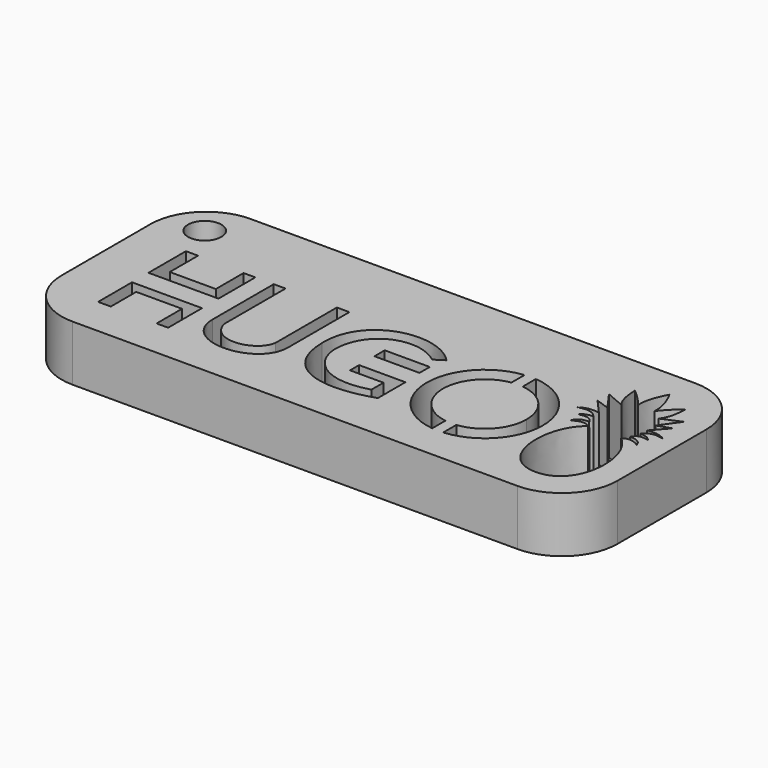
from build123d import *

# Parameters (mm, degrees)
F0_R     = 1.5
F0_W     = 3.6842799746
F0_H     = 1.051153522
F1_DEPTH = 5
F3_DEPTH = 25
F2_W     = 3.6842799746
F2_H     = 1.051153522
F4_SCALE = 1.1
F8_DEPTH = 5


with BuildPart() as f1:
    # F0 (on Top) → F1 (new body)
    with BuildSketch(Plane.XY):
        with BuildLine():
            Line((19.5023587838, 5.8855334138), (-19.8380679384, 5.8855334138))
            ThreePointArc((-19.8380679384, 5.8855334138), (-23.3736018443, 4.4210673197), (-24.8380679384, 0.8855334138))
            Line((-24.8380679384, 0.8855334138), (-24.8380679384, -9.1144665862))
            ThreePointArc((-24.8380679384, -9.1144665862), (-23.3736018443, -12.6500004921), (-19.8380679384, -14.1144665862))
            Line((-19.8380679384, -14.1144665862), (19.8321454227, -14.1144665862))
            Line((19.8321454227, -14.1144665862), (19.8321454227, -11.658272632))
            add(Edge.make_bspline(
                [(18.3578059077, -3.9089675993), (15.9339979291, -5.7451855391), (16.1109714375, -11.6508233578), (19.8321454227, -11.658272632)],
                knots=[0, 0, 0, 0, 7.8883081517, 7.8883081517, 7.8883081517, 7.8883081517], degree=3))
            add(Edge.make_bspline(
                [(18.3578059077, -3.9089675993), (18.0898513645, -3.72885447), (17.704680562, -3.4674885683), (16.8380476534, -4.0177325718)],
                knots=[0, 0, 0, 0, 1.5236452903, 1.5236452903, 1.5236452903, 1.5236452903], degree=3))
            add(Edge.make_bspline(
                [(16.8380476534, -4.0177325718), (16.9854741544, -3.645024728), (17.2194819897, -3.3108589705), (17.980273813, -3.3471628558)],
                knots=[0, 0, 0, 0, 1.3245166453, 1.3245166453, 1.3245166453, 1.3245166453], degree=3))
            add(Edge.make_bspline(
                [(17.980273813, -3.3471628558), (17.7715364844, -2.8870156966), (17.4005404115, -2.7581979521), (16.6894663125, -2.9488482978)],
                knots=[0, 0, 0, 0, 1.3508658299, 1.3508658299, 1.3508658299, 1.3508658299], degree=3))
            add(Edge.make_bspline(
                [(16.6894663125, -2.9488482978), (16.9780198485, -2.5830056984), (17.2820296139, -2.5572420564), (17.709704116, -2.5057150051)],
                knots=[0, 0, 0, 0, 1.1123184305, 1.1123184305, 1.1123184305, 1.1123184305], degree=3))
            add(Edge.make_bspline(
                [(17.709704116, -2.5057150051), (17.3335559666, -2.0625817124), (16.911033541, -1.8873894587), (15.9629341215, -2.1450251807)],
                knots=[0, 0, 0, 0, 1.7836206332, 1.7836206332, 1.7836206332, 1.7836206332], degree=3))
            add(Edge.make_bspline(
                [(15.9629341215, -2.1450251807), (16.4724756032, -1.8160737818), (16.910193488, -1.7090764595), (17.6636241376, -1.833897084)],
                knots=[0, 0, 0, 0, 1.7289150423, 1.7289150423, 1.7289150423, 1.7289150423], degree=3))
            Line((17.6636241376, -1.833897084), (16.4479874074, -0.4642672138))
            Line((16.4479874074, -0.4642672138), (17.6636241376, -0.8728023386))
            Line((17.6636241376, -0.8728023386), (16.4674408734, 0.80024614))
            Line((16.4674408734, 0.80024614), (18.1502159685, 0.0804461743))
            add(Edge.make_bspline(
                [(18.1502159685, 0.0804461743), (17.6389329135, 0.7689933409), (17.5869781524, 1.583578065), (17.5523143262, 2.3634997196)],
                knots=[0, 0, 0, 0, 2.3600465811, 2.3600465811, 2.3600465811, 2.3600465811], degree=3))
            add(Edge.make_bspline(
                [(17.5523143262, 2.3634997196), (18.1155912578, 1.9042125205), (18.6268724501, 1.3842647895), (19.0861597657, 0.7949906867)],
                knots=[0, 0, 0, 0, 2.1938328147, 2.1938328147, 2.1938328147, 2.1938328147], degree=3))
            add(Edge.make_bspline(
                [(19.0861597657, 0.7949906867), (19.0428327769, 1.834886265), (19.4855127484, 2.7450120877), (19.8321454227, 3.3949467222)],
                knots=[0, 0, 0, 0, 2.7048596982, 2.7048596982, 2.7048596982, 2.7048596982], degree=3))
            Line((19.8321454227, 3.3949467222), (19.8321454227, 5.8855334138))
            Line((19.8321454227, 5.8855334138), (19.5023587838, 5.8855334138))
        make_face()
        Polygon((-18.4758203104, -8.4118791856), (-18.4758203104, -4.9438001588), (-12.7506656572, -4.9438001588), (-12.7506656572, -8.4118791856), (-13.6949932203, -8.4118791856), (-13.6949932203, -5.8127497323), (-17.4366505817, -5.8127497323), (-17.4366505817, -8.4118791856), align=None, mode=Mode.SUBTRACT)
        with BuildLine():
            Line((-11.2475687638, 0.5051106564), (-10.28258726, 0.5051106564))
            Line((-10.28258726, 0.5051106564), (-10.28258726, -5.7747550309))
            add(Edge.make_bspline(
                [(-10.28258726, -5.7747550309), (-9.6610095352, -8.0933230929), (-6.3765929081, -7.5540901162), (-6.0863830149, -5.7747550309)],
                knots=[0, 0, 0, 0, 4.1962042451, 4.1962042451, 4.1962042451, 4.1962042451], degree=3))
            Line((-6.0863830149, -5.7747550309), (-6.0863830149, 0.5051106564))
            Line((-6.0863830149, 0.5051106564), (-5.0600701943, 0.5051106564))
            Line((-5.0600701943, 0.5051106564), (-5.0600701943, -5.7747550309))
            add(Edge.make_bspline(
                [(-11.2475687638, -5.7747550309), (-11.1742718145, -9.378020186), (-5.1037431695, -9.094146546), (-5.0600701943, -5.7747550309)],
                knots=[0, 0, 0, 0, 6.1874985695, 6.1874985695, 6.1874985695, 6.1874985695], degree=3))
            Line((-11.2475687638, -5.7747550309), (-11.2475687638, 0.5051106564))
        make_face(mode=Mode.SUBTRACT)
        Polygon((-18.4758203104, -3.2631196082), (-18.4758203104, 0.5636939313), (-17.4814509228, 0.5636939313), (-17.4814509228, -2.3290156387), (-13.7149021029, -2.3290156387), (-13.7149021029, 0.5034292699), (-12.7506656572, 0.5034292699), (-12.7506656572, -3.2631196082), align=None, mode=Mode.SUBTRACT)
        with BuildLine():
            Line((0, -5.7576037943), (0, -4.8301159404))
            Line((0, -4.8301159404), (3.7868814543, -4.8301159404))
            Line((3.7868814543, -4.8301159404), (3.7868814543, -7.6430118643))
            add(Edge.make_bspline(
                [(3.7868814543, -7.6430118643), (-0.6448045024, -9.0953717008), (-3.7148606498, -7.6815304346), (-3.7634165492, -3.8959709927)],
                knots=[0, 0, 0, 0, 8.4289569482, 8.4289569482, 8.4289569482, 8.4289569482], degree=3))
            add(Edge.make_bspline(
                [(-3.7634165492, -3.8959709927), (-3.8432804868, 0.7410292746), (1.5492066741, 1.7253720434), (3.9456789382, -0.8220763411)],
                knots=[0, 0, 0, 0, 8.2993362122, 8.2993362122, 8.2993362122, 8.2993362122], degree=3))
            Line((3.9456789382, -0.8220763411), (3.1614722684, -1.3232869096))
            add(Edge.make_bspline(
                [(-2.5977680925, -3.9639989845), (-2.4452551734, -0.6087126676), (0.9862877196, 0.4207501479), (3.1614722684, -1.3232869096)],
                knots=[0, 0, 0, 0, 6.3357880171, 6.3357880171, 6.3357880171, 6.3357880171], degree=3))
            add(Edge.make_bspline(
                [(-2.5977680925, -3.9639989845), (-2.5596399792, -6.2135658227), (-0.424457714, -7.929337211), (2.7369088493, -6.9844960235)],
                knots=[0, 0, 0, 0, 6.1304306893, 6.1304306893, 6.1304306893, 6.1304306893], degree=3))
            Line((2.7369088493, -6.9844960235), (2.7369088493, -5.7576037943))
            Line((2.7369088493, -5.7576037943), (0, -5.7576037943))
        make_face(mode=Mode.SUBTRACT)
        with Locations((-21.2343204767, 2.4730840232)):
            Circle(F0_R, mode=Mode.SUBTRACT)
        with Locations((1.8421399873, -2.7362464461)):
            Rectangle(F0_W, F0_H, mode=Mode.SUBTRACT)
        with BuildLine():
            ThreePointArc((9.8808880553, 0.7234794267), (13.0749451166, -0.7499501583), (14.3781239981, -4.0171691677))
            ThreePointArc((14.3781239981, -4.0171691677), (13.0749451166, -7.2843881771), (9.8808880553, -8.7578177622))
            ThreePointArc((9.8808880553, -8.7578177622), (9.6308880553, -8.7644051105), (9.3808880553, -8.7578177622))
            ThreePointArc((9.3808880553, -8.7578177622), (4.8836521126, -4.0171691677), (9.3808880553, 0.7234794267))
            ThreePointArc((9.3808880553, 0.7234794267), (9.6308880553, 0.730066775), (9.8808880553, 0.7234794267))
        make_face(mode=Mode.SUBTRACT)
        with BuildLine():
            Line((20.1619320616, 5.8855334138), (19.8321454227, 5.8855334138))
            Line((19.8321454227, 5.8855334138), (19.8321454227, 3.3949467222))
            add(Edge.make_bspline(
                [(20.5781310797, 0.7949906867), (20.6214580685, 1.834886265), (20.178778097, 2.7450120877), (19.8321454227, 3.3949467222)],
                knots=[0, 0, 0, 0, 2.7048596982, 2.7048596982, 2.7048596982, 2.7048596982], degree=3))
            add(Edge.make_bspline(
                [(22.1119765192, 2.3634997196), (21.5486995876, 1.9042125205), (21.0374183953, 1.3842647895), (20.5781310797, 0.7949906867)],
                knots=[0, 0, 0, 0, 2.1938328147, 2.1938328147, 2.1938328147, 2.1938328147], degree=3))
            add(Edge.make_bspline(
                [(21.5140748769, 0.0804461743), (22.0253579319, 0.7689933409), (22.077312693, 1.583578065), (22.1119765192, 2.3634997196)],
                knots=[0, 0, 0, 0, 2.3600465811, 2.3600465811, 2.3600465811, 2.3600465811], degree=3))
            Line((21.5140748769, 0.0804461743), (23.196849972, 0.80024614))
            Line((23.196849972, 0.80024614), (22.0006667078, -0.8728023386))
            Line((22.0006667078, -0.8728023386), (23.2163034379, -0.4642672138))
            Line((23.2163034379, -0.4642672138), (22.0006667078, -1.833897084))
            add(Edge.make_bspline(
                [(23.7013567239, -2.1450251807), (23.1918152422, -1.8160737818), (22.7540973574, -1.7090764595), (22.0006667078, -1.833897084)],
                knots=[0, 0, 0, 0, 1.7289150423, 1.7289150423, 1.7289150423, 1.7289150423], degree=3))
            add(Edge.make_bspline(
                [(21.9545867294, -2.5057150051), (22.3307348788, -2.0625817124), (22.7532573044, -1.8873894587), (23.7013567239, -2.1450251807)],
                knots=[0, 0, 0, 0, 1.7836206332, 1.7836206332, 1.7836206332, 1.7836206332], degree=3))
            add(Edge.make_bspline(
                [(22.9748245329, -2.9488482978), (22.6862709969, -2.5830056984), (22.3822612315, -2.5572420564), (21.9545867294, -2.5057150051)],
                knots=[0, 0, 0, 0, 1.1123184305, 1.1123184305, 1.1123184305, 1.1123184305], degree=3))
            add(Edge.make_bspline(
                [(21.6840170324, -3.3471628558), (21.892754361, -2.8870156966), (22.2637504339, -2.7581979521), (22.9748245329, -2.9488482978)],
                knots=[0, 0, 0, 0, 1.3508658299, 1.3508658299, 1.3508658299, 1.3508658299], degree=3))
            add(Edge.make_bspline(
                [(22.826243192, -4.0177325718), (22.678816691, -3.645024728), (22.4448088557, -3.3108589705), (21.6840170324, -3.3471628558)],
                knots=[0, 0, 0, 0, 1.3245166453, 1.3245166453, 1.3245166453, 1.3245166453], degree=3))
            add(Edge.make_bspline(
                [(21.3064849377, -3.9089675993), (21.5744394809, -3.72885447), (21.9596102834, -3.4674885683), (22.826243192, -4.0177325718)],
                knots=[0, 0, 0, 0, 1.5236452903, 1.5236452903, 1.5236452903, 1.5236452903], degree=3))
            add(Edge.make_bspline(
                [(21.3064849377, -3.9089675993), (23.7302929163, -5.7451855391), (23.5533194079, -11.6508233578), (19.8321454227, -11.658272632)],
                knots=[0, 0, 0, 0, 7.8883081517, 7.8883081517, 7.8883081517, 7.8883081517], degree=3))
            Line((19.8321454227, -11.658272632), (19.8321454227, -14.1144665862))
            Line((19.8321454227, -14.1144665862), (20.1619320616, -14.1144665862))
            ThreePointArc((20.1619320616, -14.1144665862), (23.6974659676, -12.6500004921), (25.1619320616, -9.1144665862))
            Line((25.1619320616, -9.1144665862), (25.1619320616, 0.8855334138))
            ThreePointArc((25.1619320616, 0.8855334138), (23.6974659676, 4.4210673197), (20.1619320616, 5.8855334138))
        make_face()
        Polygon((-17.4814509228, 0.5636939313), (-18.4758203104, 0.5636939313), (-18.4758203104, -3.2631196082), (-12.7506656572, -3.2631196082), (-12.7506656572, 0.5034292699), (-13.7149021029, 0.5034292699), (-13.7149021029, -2.3290156387), (-17.4814509228, -2.3290156387), align=None)
        Polygon((-12.7506656572, -4.9438001588), (-18.4758203104, -4.9438001588), (-18.4758203104, -8.4118791856), (-17.4366505817, -8.4118791856), (-17.4366505817, -5.8127497323), (-13.6949932203, -5.8127497323), (-13.6949932203, -8.4118791856), (-12.7506656572, -8.4118791856), align=None)
        with BuildLine():
            Line((-10.28258726, -5.7747550309), (-10.28258726, 0.5051106564))
            Line((-10.28258726, 0.5051106564), (-11.2475687638, 0.5051106564))
            Line((-11.2475687638, 0.5051106564), (-11.2475687638, -5.7747550309))
            add(Edge.make_bspline(
                [(-11.2475687638, -5.7747550309), (-11.1742718145, -9.378020186), (-5.1037431695, -9.094146546), (-5.0600701943, -5.7747550309)],
                knots=[0, 0, 0, 0, 6.1874985695, 6.1874985695, 6.1874985695, 6.1874985695], degree=3))
            Line((-5.0600701943, -5.7747550309), (-5.0600701943, 0.5051106564))
            Line((-5.0600701943, 0.5051106564), (-6.0863830149, 0.5051106564))
            Line((-6.0863830149, 0.5051106564), (-6.0863830149, -5.7747550309))
            add(Edge.make_bspline(
                [(-10.28258726, -5.7747550309), (-9.6610095352, -8.0933230929), (-6.3765929081, -7.5540901162), (-6.0863830149, -5.7747550309)],
                knots=[0, 0, 0, 0, 4.1962042451, 4.1962042451, 4.1962042451, 4.1962042451], degree=3))
        make_face()
        with Locations((1.8421399873, -2.7362464461)):
            Rectangle(F0_W, F0_H)
        with BuildLine():
            Line((3.7868814543, -4.8301159404), (0, -4.8301159404))
            Line((0, -4.8301159404), (0, -5.7576037943))
            Line((0, -5.7576037943), (2.7369088493, -5.7576037943))
            Line((2.7369088493, -5.7576037943), (2.7369088493, -6.9844960235))
            add(Edge.make_bspline(
                [(-2.5977680925, -3.9639989845), (-2.5596399792, -6.2135658227), (-0.424457714, -7.929337211), (2.7369088493, -6.9844960235)],
                knots=[0, 0, 0, 0, 6.1304306893, 6.1304306893, 6.1304306893, 6.1304306893], degree=3))
            add(Edge.make_bspline(
                [(-2.5977680925, -3.9639989845), (-2.4452551734, -0.6087126676), (0.9862877196, 0.4207501479), (3.1614722684, -1.3232869096)],
                knots=[0, 0, 0, 0, 6.3357880171, 6.3357880171, 6.3357880171, 6.3357880171], degree=3))
            Line((3.1614722684, -1.3232869096), (3.9456789382, -0.8220763411))
            add(Edge.make_bspline(
                [(-3.7634165492, -3.8959709927), (-3.8432804868, 0.7410292746), (1.5492066741, 1.7253720434), (3.9456789382, -0.8220763411)],
                knots=[0, 0, 0, 0, 8.2993362122, 8.2993362122, 8.2993362122, 8.2993362122], degree=3))
            add(Edge.make_bspline(
                [(3.7868814543, -7.6430118643), (-0.6448045024, -9.0953717008), (-3.7148606498, -7.6815304346), (-3.7634165492, -3.8959709927)],
                knots=[0, 0, 0, 0, 8.4289569482, 8.4289569482, 8.4289569482, 8.4289569482], degree=3))
            Line((3.7868814543, -7.6430118643), (3.7868814543, -4.8301159404))
        make_face()
        with BuildLine():
            ThreePointArc((9.8808880553, -8.7578177622), (13.0749451166, -7.2843881771), (14.3781239981, -4.0171691677))
            ThreePointArc((14.3781239981, -4.0171691677), (13.0749451166, -0.7499501583), (9.8808880553, 0.7234794267))
            Line((9.8808880553, 0.7234794267), (9.8808880553, -0.6084652765))
            ThreePointArc((9.8808880553, -0.6084652765), (12.1345081388, -1.6904442815), (13.0487473588, -4.0171691677))
            ThreePointArc((13.0487473588, -4.0171691677), (12.1345081388, -6.343894054), (9.8808880553, -7.425873059))
            Line((9.8808880553, -7.425873059), (9.8808880553, -8.7578177622))
        make_face()
        with BuildLine():
            Line((9.8808880553, -0.6084652765), (9.8808880553, 0.7234794267))
            ThreePointArc((9.8808880553, 0.7234794267), (9.6308880553, 0.730066775), (9.3808880553, 0.7234794267))
            Line((9.3808880553, 0.7234794267), (9.3808880553, -0.6084652765))
            ThreePointArc((9.3808880553, -0.6084652765), (9.6308880553, -0.5993098643), (9.8808880553, -0.6084652765))
        make_face()
        with BuildLine():
            ThreePointArc((9.3808880553, -8.7578177622), (9.6308880553, -8.7644051105), (9.8808880553, -8.7578177622))
            Line((9.8808880553, -8.7578177622), (9.8808880553, -7.425873059))
            ThreePointArc((9.8808880553, -7.425873059), (9.6308880553, -7.4350284712), (9.3808880553, -7.425873059))
            Line((9.3808880553, -7.425873059), (9.3808880553, -8.7578177622))
        make_face()
        with BuildLine():
            Line((9.3808880553, -0.6084652765), (9.3808880553, 0.7234794267))
            ThreePointArc((9.3808880553, 0.7234794267), (4.8836521126, -4.0171691677), (9.3808880553, -8.7578177622))
            Line((9.3808880553, -8.7578177622), (9.3808880553, -7.425873059))
            ThreePointArc((9.3808880553, -7.425873059), (6.2130287519, -4.0171691677), (9.3808880553, -0.6084652765))
        make_face()
        with BuildLine():
            ThreePointArc((13.0487473588, -4.0171691677), (12.1345081388, -1.6904442815), (9.8808880553, -0.6084652765))
            ThreePointArc((9.8808880553, -0.6084652765), (9.6308880553, -0.5993098643), (9.3808880553, -0.6084652765))
            ThreePointArc((9.3808880553, -0.6084652765), (6.2130287519, -4.0171691677), (9.3808880553, -7.425873059))
            ThreePointArc((9.3808880553, -7.425873059), (9.6308880553, -7.4350284712), (9.8808880553, -7.425873059))
            ThreePointArc((9.8808880553, -7.425873059), (12.1345081388, -6.343894054), (13.0487473588, -4.0171691677))
        make_face()
    extrude(amount=F1_DEPTH)


with BuildPart() as f3:
    # F2 (on face) → F3 (new body)
    with BuildSketch(Plane.XY.offset(5)):
        Polygon((-13.6949932203, -5.8127497323), (-13.6949932203, -8.4118791856), (-12.7506656572, -8.4118791856), (-12.7506656572, -4.9438001588), (-18.4758203104, -4.9438001588), (-18.4758203104, -8.4118791856), (-17.4366505817, -8.4118791856), (-17.4366505817, -5.8127497323), align=None)
    extrude(amount=F3_DEPTH)


with BuildPart() as f3b:
    # F2 (on face) → F3, piece 2 (new body)
    with BuildSketch(Plane.XY.offset(5)):
        with BuildLine():
            Line((3.7868814543, -7.6430118643), (3.7868814543, -4.8301159404))
            Line((3.7868814543, -4.8301159404), (0, -4.8301159404))
            Line((0, -4.8301159404), (0, -5.7576037943))
            Line((0, -5.7576037943), (2.7369088493, -5.7576037943))
            Line((2.7369088493, -5.7576037943), (2.7369088493, -6.9844960235))
            add(Edge.make_bspline(
                [(-2.5977680925, -3.9639989845), (-2.5596399792, -6.2135658227), (-0.424457714, -7.929337211), (2.7369088493, -6.9844960235)],
                knots=[0, 0, 0, 0, 1, 1, 1, 1], degree=3))
            add(Edge.make_bspline(
                [(-2.5977680925, -3.9639989845), (-2.4452551734, -0.6087126676), (0.9862877196, 0.4207501479), (3.1614722684, -1.3232869096)],
                knots=[0, 0, 0, 0, 1, 1, 1, 1], degree=3))
            Line((3.1614722684, -1.3232869096), (3.9456789382, -0.8220763411))
            add(Edge.make_bspline(
                [(-3.7634165492, -3.8959709927), (-3.8432804868, 0.7410292746), (1.5492066741, 1.7253720434), (3.9456789382, -0.8220763411)],
                knots=[0, 0, 0, 0, 1, 1, 1, 1], degree=3))
            add(Edge.make_bspline(
                [(3.7868814543, -7.6430118643), (-0.6448045024, -9.0953717008), (-3.7148606498, -7.6815304346), (-3.7634165492, -3.8959709927)],
                knots=[0, 0, 0, 0, 1, 1, 1, 1], degree=3))
        make_face()
    extrude(amount=F3_DEPTH)


with BuildPart() as f3c:
    # F2 (on face) → F3, piece 3 (new body)
    with BuildSketch(Plane.XY.offset(5)):
        with BuildLine():
            Line((-10.28258726, -5.7747550309), (-10.28258726, 0.5051106564))
            Line((-10.28258726, 0.5051106564), (-11.2475687638, 0.5051106564))
            Line((-11.2475687638, 0.5051106564), (-11.2475687638, -5.7747550309))
            add(Edge.make_bspline(
                [(-11.2475687638, -5.7747550309), (-11.1742718145, -9.378020186), (-5.1037431695, -9.094146546), (-5.0600701943, -5.7747550309)],
                knots=[0, 0, 0, 0, 1, 1, 1, 1], degree=3))
            Line((-5.0600701943, -5.7747550309), (-5.0600701943, 0.5051106564))
            Line((-5.0600701943, 0.5051106564), (-6.0863830149, 0.5051106564))
            Line((-6.0863830149, 0.5051106564), (-6.0863830149, -5.7747550309))
            add(Edge.make_bspline(
                [(-10.28258726, -5.7747550309), (-9.6610095352, -8.0933230929), (-6.3765929081, -7.5540901162), (-6.0863830149, -5.7747550309)],
                knots=[0, 0, 0, 0, 1, 1, 1, 1], degree=3))
        make_face()
    extrude(amount=F3_DEPTH)


with BuildPart() as f3d:
    # F2 (on face) → F3, piece 4 (new body)
    with BuildSketch(Plane.XY.offset(5)):
        with BuildLine():
            ThreePointArc((9.8808880553, -8.7578177622), (13.0749451166, -7.2843881771), (14.3781239981, -4.0171691677))
            ThreePointArc((14.3781239981, -4.0171691677), (13.0749451166, -0.7499501583), (9.8808880553, 0.7234794267))
            Line((9.8808880553, 0.7234794267), (9.8808880553, -0.6084652765))
            ThreePointArc((9.8808880553, -0.6084652765), (12.1345081388, -1.6904442815), (13.0487473588, -4.0171691677))
            ThreePointArc((13.0487473588, -4.0171691677), (12.1345081388, -6.343894054), (9.8808880553, -7.425873059))
            Line((9.8808880553, -7.425873059), (9.8808880553, -8.7578177622))
        make_face()
        with BuildLine():
            Line((9.8808880553, -0.6084652765), (9.8808880553, 0.7234794267))
            ThreePointArc((9.8808880553, 0.7234794267), (9.6308880553, 0.730066775), (9.3808880553, 0.7234794267))
            Line((9.3808880553, 0.7234794267), (9.3808880553, -0.6084652765))
            ThreePointArc((9.3808880553, -0.6084652765), (9.6308880553, -0.5993098643), (9.8808880553, -0.6084652765))
        make_face()
        with BuildLine():
            ThreePointArc((9.3808880553, -8.7578177622), (9.6308880553, -8.7644051105), (9.8808880553, -8.7578177622))
            Line((9.8808880553, -8.7578177622), (9.8808880553, -7.425873059))
            ThreePointArc((9.8808880553, -7.425873059), (9.6308880553, -7.4350284712), (9.3808880553, -7.425873059))
            Line((9.3808880553, -7.425873059), (9.3808880553, -8.7578177622))
        make_face()
        with BuildLine():
            Line((9.3808880553, -0.6084652765), (9.3808880553, 0.7234794267))
            ThreePointArc((9.3808880553, 0.7234794267), (4.8836521126, -4.0171691677), (9.3808880553, -8.7578177622))
            Line((9.3808880553, -8.7578177622), (9.3808880553, -7.425873059))
            ThreePointArc((9.3808880553, -7.425873059), (6.2130287519, -4.0171691677), (9.3808880553, -0.6084652765))
        make_face()
    extrude(amount=F3_DEPTH)


with BuildPart() as f3e:
    # F2 (on face) → F3, piece 5 (new body)
    with BuildSketch(Plane.XY.offset(5)):
        with Locations((1.8421399873, -2.7362464461)):
            Rectangle(F2_W, F2_H)
    extrude(amount=F3_DEPTH)


with BuildPart() as f3f:
    # F2 (on face) → F3, piece 6 (new body)
    with BuildSketch(Plane.XY.offset(5)):
        Polygon((-13.7149021029, 0.5034292699), (-13.7149021029, -2.3290156387), (-17.4814509228, -2.3290156387), (-17.4814509228, 0.5636939313), (-18.4758203104, 0.5636939313), (-18.4758203104, -3.2631196082), (-12.7506656572, -3.2631196082), (-12.7506656572, 0.5034292699), align=None)
    extrude(amount=F3_DEPTH)


with BuildPart() as f3_1:
    # F4: moved
    add(f3.part.scale(F4_SCALE))


with BuildPart() as f3b_1:
    # F4: moved
    add(f3b.part.scale(F4_SCALE))


with BuildPart() as f3c_1:
    # F4: moved
    add(f3c.part.scale(F4_SCALE))


with BuildPart() as f3d_1:
    # F4: moved
    add(f3d.part.scale(F4_SCALE))


with BuildPart() as f3e_1:
    # F4: moved
    add(f3e.part.scale(F4_SCALE))


with BuildPart() as f3f_1:
    # F4: moved
    add(f3f.part.scale(F4_SCALE))


with BuildPart() as f3_2:
    # F5: moved
    add(f3_1.part.moved(Location((0, -1.4, -11))))


with BuildPart() as f3b_2:
    # F5: moved
    add(f3b_1.part.moved(Location((0, -1.4, -11))))


with BuildPart() as f3c_2:
    # F5: moved
    add(f3c_1.part.moved(Location((0, -1.4, -11))))


with BuildPart() as f3d_2:
    # F5: moved
    add(f3d_1.part.moved(Location((0, -1.4, -11))))


with BuildPart() as f3e_2:
    # F5: moved
    add(f3e_1.part.moved(Location((0, -1.4, -11))))


with BuildPart() as f3f_2:
    # F5: moved
    add(f3f_1.part.moved(Location((0, -1.4, -11))))


with BuildPart() as f1_1:
    add(f1.part)

    # F6: cut F3, F3b, F3c, F3d, F3e, F3f
    add(f3_2.part, mode=Mode.SUBTRACT)
    add(f3b_2.part, mode=Mode.SUBTRACT)
    add(f3c_2.part, mode=Mode.SUBTRACT)
    add(f3d_2.part, mode=Mode.SUBTRACT)
    add(f3e_2.part, mode=Mode.SUBTRACT)
    add(f3f_2.part, mode=Mode.SUBTRACT)

    # F7 (on face) → F8 (join, through all)
    with BuildSketch(Plane.XY.offset(5)):
        with BuildLine():
            Line((11.0160996318, 2.141247374), (10.0160996318, 2.1032726459))
            Line((10.0160996318, 2.1032726459), (10.0160996318, -2.1039176873))
            ThreePointArc((10.0160996318, -2.1039176873), (10.5154013556, -2.0600620431), (11.0160996318, -2.0830134086))
            Line((11.0160996318, -2.0830134086), (11.0160996318, 2.141247374))
        make_face()
        with BuildLine():
            ThreePointArc((11.0160996318, -9.5547587604), (10.5154013556, -9.5777101259), (10.0160996318, -9.5338544817))
            Line((10.0160996318, -9.5338544817), (10.0160996318, -11.3756301854))
            Line((10.0160996318, -11.3756301854), (11.0160996318, -11.3756301854))
            Line((11.0160996318, -11.3756301854), (11.0160996318, -9.5547587604))
        make_face()
    extrude(amount=-F8_DEPTH)


solid = f1_1.part
